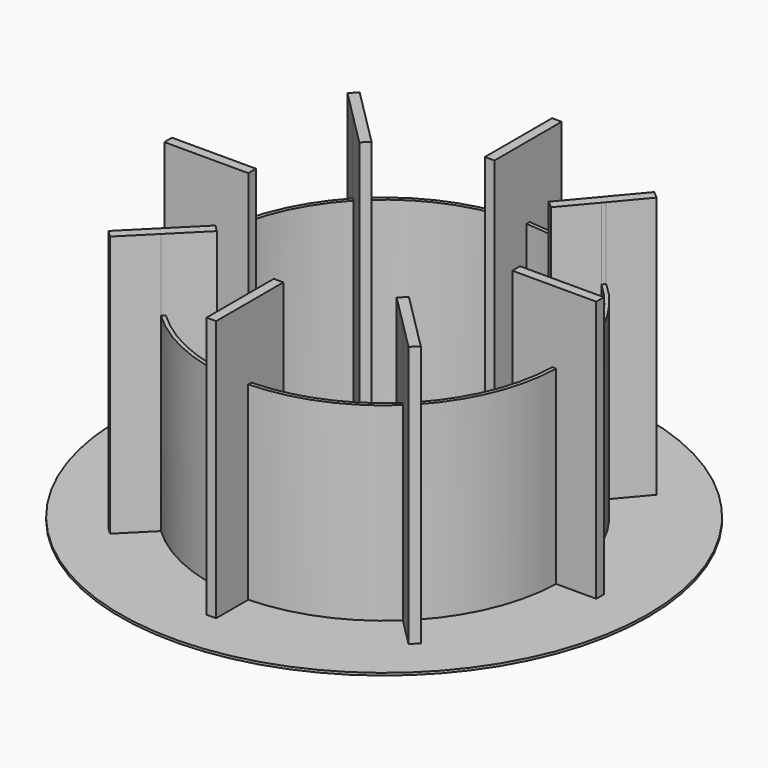
from build123d import *

# Parameters (mm, degrees)
F0_R     = 110
F1_DEPTH = 1
F0_R_2   = 7.5
F2_DEPTH = 110
F3_DEPTH = 80


with BuildPart() as f1:
    # F0 (on Top) → F1 (new body)
    with BuildSketch(Plane.XY):
        Circle(F0_R)
        with BuildLine():
            Line((-90, 2), (-73.2727097902, 2))
            ThreePointArc((-73.2727097902, 2), (-67.7203697331, 28.0506955924), (-53.2258435309, 50.3974164062))
            Line((-53.2258435309, 50.3974164062), (-65.0538238692, 62.2253967444))
            Line((-65.0538238692, 62.2253967444), (-62.2253967444, 65.0538238692))
            Line((-62.2253967444, 65.0538238692), (-50.3974164062, 53.2258435309))
            ThreePointArc((-50.3974164062, 53.2258435309), (-28.0506955924, 67.7203697331), (-2, 73.2727097902))
            Line((-2, 73.2727097902), (-2, 90))
            Line((-2, 90), (2, 90))
            Line((2, 90), (2, 73.2727097902))
            ThreePointArc((2, 73.2727097902), (25.1459027822, 68.8518233111), (45.6930285955, 57.3152435027))
            Line((45.6930285955, 57.3152435027), (56.4733154171, 70.105382431))
            Line((56.4733154171, 70.105382431), (59.5318237034, 67.5274904506))
            Line((59.5318237034, 67.5274904506), (48.7515368817, 54.7373515223))
            ThreePointArc((48.7515368817, 54.7373515223), (66.4664295367, 30.904752784), (73.2727097902, 2))
            Line((73.2727097902, 2), (90, 2))
            Line((90, 2), (90, -2))
            Line((90, -2), (73.2727097902, -2))
            ThreePointArc((73.2727097902, -2), (67.7203697331, -28.0506955924), (53.2258435309, -50.3974164062))
            Line((53.2258435309, -50.3974164062), (65.0538238692, -62.2253967444))
            Line((65.0538238692, -62.2253967444), (62.2253967444, -65.0538238692))
            Line((62.2253967444, -65.0538238692), (50.3974164062, -53.2258435309))
            ThreePointArc((50.3974164062, -53.2258435309), (28.0506955924, -67.7203697331), (2, -73.2727097902))
            Line((2, -73.2727097902), (2, -90))
            Line((2, -90), (-2, -90))
            Line((-2, -90), (-2, -73.2727097902))
            ThreePointArc((-2, -73.2727097902), (-28.0506955924, -67.7203697331), (-50.3974164062, -53.2258435309))
            Line((-50.3974164062, -53.2258435309), (-62.2253967444, -65.0538238692))
            Line((-62.2253967444, -65.0538238692), (-65.0538238692, -62.2253967444))
            Line((-65.0538238692, -62.2253967444), (-53.2258435309, -50.3974164062))
            ThreePointArc((-53.2258435309, -50.3974164062), (-67.7203697331, -28.0506955924), (-73.2727097902, -2))
            Line((-73.2727097902, -2), (-90, -2))
            Line((-90, -2), (-90, 2))
        make_face(mode=Mode.SUBTRACT)
    extrude(amount=F1_DEPTH)



with BuildPart() as f1b:
    # F0 (on Top) → F1, piece 2 (new body)
    with BuildSketch(Plane.XY):
        with BuildLine():
            Line((-71.6721005692, 2), (-55, 2))
            Line((-55, 2), (-55, -2))
            Line((-55, -2), (-71.6721005692, -2))
            ThreePointArc((-71.6721005692, -2), (-66.2421624811, -27.4384021006), (-52.0940418967, -49.265614772))
            Line((-52.0940418967, -49.265614772), (-40.3050865276, -37.4766594029))
            Line((-40.3050865276, -37.4766594029), (-37.4766594029, -40.3050865276))
            Line((-37.4766594029, -40.3050865276), (-49.265614772, -52.0940418967))
            ThreePointArc((-49.265614772, -52.0940418967), (-27.4384021006, -66.2421624811), (-2, -71.6721005692))
            Line((-2, -71.6721005692), (-2, -55))
            Line((-2, -55), (2, -55))
            Line((2, -55), (2, -71.6721005692))
            ThreePointArc((2, -71.6721005692), (27.4384021006, -66.2421624811), (49.265614772, -52.0940418967))
            Line((49.265614772, -52.0940418967), (37.4766594029, -40.3050865276))
            Line((37.4766594029, -40.3050865276), (40.3050865276, -37.4766594029))
            Line((40.3050865276, -37.4766594029), (52.0940418967, -49.265614772))
            ThreePointArc((52.0940418967, -49.265614772), (66.2421624811, -27.4384021006), (71.6721005692, -2))
            Line((71.6721005692, -2), (55, -2))
            Line((55, -2), (55, 2))
            Line((55, 2), (71.6721005692, 2))
            ThreePointArc((71.6721005692, 2), (65.0155934213, 30.2301606359), (47.719987463, 53.5134823809))
            Line((47.719987463, 53.5134823809), (36.9752688744, 40.7655429458))
            Line((36.9752688744, 40.7655429458), (33.9167605881, 43.3434349263))
            Line((33.9167605881, 43.3434349263), (44.6614791768, 56.0913743613))
            ThreePointArc((44.6614791768, 56.0913743613), (24.597015409, 67.3489185731), (2, 71.6721005692))
            Line((2, 71.6721005692), (2, 55))
            Line((2, 55), (-2, 55))
            Line((-2, 55), (-2, 71.6721005692))
            ThreePointArc((-2, 71.6721005692), (-27.4384021006, 66.2421624811), (-49.265614772, 52.0940418967))
            Line((-49.265614772, 52.0940418967), (-37.4766594029, 40.3050865276))
            Line((-37.4766594029, 40.3050865276), (-40.3050865276, 37.4766594029))
            Line((-40.3050865276, 37.4766594029), (-52.0940418967, 49.265614772))
            ThreePointArc((-52.0940418967, 49.265614772), (-66.2421624811, 27.4384021006), (-71.6721005692, 2))
        make_face()
        Circle(F0_R_2, mode=Mode.SUBTRACT)
    extrude(amount=F1_DEPTH)


with BuildPart() as f1_1:
    add(f1.part)

    add(f1b.part)  # F2 merges F1b
    # F0 (on Top) → F2 (join)
    with BuildSketch(Plane.XY):
        with BuildLine():
            Line((-55, -2), (-55, 2))
            Line((-55, 2), (-71.6721005692, 2))
            ThreePointArc((-71.6721005692, 2), (-71.7, 0), (-71.6721005692, -2))
            Line((-71.6721005692, -2), (-55, -2))
        make_face()
        with BuildLine():
            ThreePointArc((-71.6721005692, -2), (-71.7, 0), (-71.6721005692, 2))
            Line((-71.6721005692, 2), (-73.2727097902, 2))
            ThreePointArc((-73.2727097902, 2), (-73.3, 0), (-73.2727097902, -2))
            Line((-73.2727097902, -2), (-71.6721005692, -2))
        make_face()
        with BuildLine():
            ThreePointArc((-73.2727097902, -2), (-73.3, 0), (-73.2727097902, 2))
            Line((-73.2727097902, 2), (-90, 2))
            Line((-90, 2), (-90, -2))
            Line((-90, -2), (-73.2727097902, -2))
        make_face()
        with BuildLine():
            ThreePointArc((-49.265614772, 52.0940418967), (-50.6995562111, 50.6995562111), (-52.0940418967, 49.265614772))
            Line((-52.0940418967, 49.265614772), (-40.3050865276, 37.4766594029))
            Line((-40.3050865276, 37.4766594029), (-37.4766594029, 40.3050865276))
            Line((-37.4766594029, 40.3050865276), (-49.265614772, 52.0940418967))
        make_face()
        with BuildLine():
            Line((-53.2258435309, 50.3974164062), (-52.0940418967, 49.265614772))
            ThreePointArc((-52.0940418967, 49.265614772), (-50.6995562111, 50.6995562111), (-49.265614772, 52.0940418967))
            Line((-49.265614772, 52.0940418967), (-50.3974164062, 53.2258435309))
            ThreePointArc((-50.3974164062, 53.2258435309), (-51.830927061, 51.830927061), (-53.2258435309, 50.3974164062))
        make_face()
        with BuildLine():
            Line((-65.0538238692, 62.2253967444), (-53.2258435309, 50.3974164062))
            ThreePointArc((-53.2258435309, 50.3974164062), (-51.830927061, 51.830927061), (-50.3974164062, 53.2258435309))
            Line((-50.3974164062, 53.2258435309), (-62.2253967444, 65.0538238692))
            Line((-62.2253967444, 65.0538238692), (-65.0538238692, 62.2253967444))
        make_face()
        with BuildLine():
            ThreePointArc((2, 71.6721005692), (0, 71.7), (-2, 71.6721005692))
            Line((-2, 71.6721005692), (-2, 55))
            Line((-2, 55), (2, 55))
            Line((2, 55), (2, 71.6721005692))
        make_face()
        with BuildLine():
            Line((-2, 73.2727097902), (-2, 71.6721005692))
            ThreePointArc((-2, 71.6721005692), (0, 71.7), (2, 71.6721005692))
            Line((2, 71.6721005692), (2, 73.2727097902))
            ThreePointArc((2, 73.2727097902), (0, 73.3), (-2, 73.2727097902))
        make_face()
        with BuildLine():
            Line((-2, 90), (-2, 73.2727097902))
            ThreePointArc((-2, 73.2727097902), (0, 73.3), (2, 73.2727097902))
            Line((2, 73.2727097902), (2, 90))
            Line((2, 90), (-2, 90))
        make_face()
        with BuildLine():
            ThreePointArc((47.719987463, 53.5134823809), (46.2087137496, 54.8237610312), (44.6614791768, 56.0913743613))
            Line((44.6614791768, 56.0913743613), (33.9167605881, 43.3434349263))
            Line((33.9167605881, 43.3434349263), (36.9752688744, 40.7655429458))
            Line((36.9752688744, 40.7655429458), (47.719987463, 53.5134823809))
        make_face()
        with BuildLine():
            Line((45.6930285955, 57.3152435027), (44.6614791768, 56.0913743613))
            ThreePointArc((44.6614791768, 56.0913743613), (46.2087137496, 54.8237610312), (47.719987463, 53.5134823809))
            Line((47.719987463, 53.5134823809), (48.7515368817, 54.7373515223))
            ThreePointArc((48.7515368817, 54.7373515223), (47.2398705418, 56.0471643457), (45.6930285955, 57.3152435027))
        make_face()
        with BuildLine():
            Line((56.4733154171, 70.105382431), (45.6930285955, 57.3152435027))
            ThreePointArc((45.6930285955, 57.3152435027), (47.2398705418, 56.0471643457), (48.7515368817, 54.7373515223))
            Line((48.7515368817, 54.7373515223), (59.5318237034, 67.5274904506))
            Line((59.5318237034, 67.5274904506), (56.4733154171, 70.105382431))
        make_face()
        with BuildLine():
            ThreePointArc((71.7, 0), (71.693024803, 1.0000972925), (71.6721005692, 2))
            Line((71.6721005692, 2), (55, 2))
            Line((55, 2), (55, -2))
            Line((55, -2), (71.6721005692, -2))
            ThreePointArc((71.6721005692, -2), (71.693024803, -1.0000972925), (71.7, 0))
        make_face()
        with BuildLine():
            Line((73.2727097902, 2), (71.6721005692, 2))
            ThreePointArc((71.6721005692, 2), (71.693024803, 1.0000972925), (71.7, 0))
            ThreePointArc((71.7, 0), (71.693024803, -1.0000972925), (71.6721005692, -2))
            Line((71.6721005692, -2), (73.2727097902, -2))
            ThreePointArc((73.2727097902, -2), (73.29317713, -1.0000930901), (73.3, 0))
            ThreePointArc((73.3, 0), (73.29317713, 1.0000930901), (73.2727097902, 2))
        make_face()
        with BuildLine():
            Line((90, 2), (73.2727097902, 2))
            ThreePointArc((73.2727097902, 2), (73.29317713, 1.0000930901), (73.3, 0))
            ThreePointArc((73.3, 0), (73.29317713, -1.0000930901), (73.2727097902, -2))
            Line((73.2727097902, -2), (90, -2))
            Line((90, -2), (90, 2))
        make_face()
        with BuildLine():
            Line((37.4766594029, -40.3050865276), (49.265614772, -52.0940418967))
            ThreePointArc((49.265614772, -52.0940418967), (50.6995562111, -50.6995562111), (52.0940418967, -49.265614772))
            Line((52.0940418967, -49.265614772), (40.3050865276, -37.4766594029))
            Line((40.3050865276, -37.4766594029), (37.4766594029, -40.3050865276))
        make_face()
        with BuildLine():
            ThreePointArc((52.0940418967, -49.265614772), (50.6995562111, -50.6995562111), (49.265614772, -52.0940418967))
            Line((49.265614772, -52.0940418967), (50.3974164062, -53.2258435309))
            ThreePointArc((50.3974164062, -53.2258435309), (51.830927061, -51.830927061), (53.2258435309, -50.3974164062))
            Line((53.2258435309, -50.3974164062), (52.0940418967, -49.265614772))
        make_face()
        with BuildLine():
            ThreePointArc((53.2258435309, -50.3974164062), (51.830927061, -51.830927061), (50.3974164062, -53.2258435309))
            Line((50.3974164062, -53.2258435309), (62.2253967444, -65.0538238692))
            Line((62.2253967444, -65.0538238692), (65.0538238692, -62.2253967444))
            Line((65.0538238692, -62.2253967444), (53.2258435309, -50.3974164062))
        make_face()
        with BuildLine():
            Line((-2, -55), (-2, -71.6721005692))
            ThreePointArc((-2, -71.6721005692), (0, -71.7), (2, -71.6721005692))
            Line((2, -71.6721005692), (2, -55))
            Line((2, -55), (-2, -55))
        make_face()
        with BuildLine():
            ThreePointArc((2, -71.6721005692), (0, -71.7), (-2, -71.6721005692))
            Line((-2, -71.6721005692), (-2, -73.2727097902))
            ThreePointArc((-2, -73.2727097902), (0, -73.3), (2, -73.2727097902))
            Line((2, -73.2727097902), (2, -71.6721005692))
        make_face()
        with BuildLine():
            ThreePointArc((2, -73.2727097902), (0, -73.3), (-2, -73.2727097902))
            Line((-2, -73.2727097902), (-2, -90))
            Line((-2, -90), (2, -90))
            Line((2, -90), (2, -73.2727097902))
        make_face()
        with BuildLine():
            Line((-40.3050865276, -37.4766594029), (-52.0940418967, -49.265614772))
            ThreePointArc((-52.0940418967, -49.265614772), (-50.6995562111, -50.6995562111), (-49.265614772, -52.0940418967))
            Line((-49.265614772, -52.0940418967), (-37.4766594029, -40.3050865276))
            Line((-37.4766594029, -40.3050865276), (-40.3050865276, -37.4766594029))
        make_face()
        with BuildLine():
            ThreePointArc((-49.265614772, -52.0940418967), (-50.6995562111, -50.6995562111), (-52.0940418967, -49.265614772))
            Line((-52.0940418967, -49.265614772), (-53.2258435309, -50.3974164062))
            ThreePointArc((-53.2258435309, -50.3974164062), (-51.830927061, -51.830927061), (-50.3974164062, -53.2258435309))
            Line((-50.3974164062, -53.2258435309), (-49.265614772, -52.0940418967))
        make_face()
        with BuildLine():
            ThreePointArc((-50.3974164062, -53.2258435309), (-51.830927061, -51.830927061), (-53.2258435309, -50.3974164062))
            Line((-53.2258435309, -50.3974164062), (-65.0538238692, -62.2253967444))
            Line((-65.0538238692, -62.2253967444), (-62.2253967444, -65.0538238692))
            Line((-62.2253967444, -65.0538238692), (-50.3974164062, -53.2258435309))
        make_face()
    extrude(amount=F2_DEPTH)

    # F0 (on Top) → F3 (join)
    with BuildSketch(Plane.XY):
        with BuildLine():
            Line((-73.2727097902, 2), (-71.6721005692, 2))
            ThreePointArc((-71.6721005692, 2), (-66.2421624811, 27.4384021006), (-52.0940418967, 49.265614772))
            Line((-52.0940418967, 49.265614772), (-53.2258435309, 50.3974164062))
            ThreePointArc((-53.2258435309, 50.3974164062), (-67.7203697331, 28.0506955924), (-73.2727097902, 2))
        make_face()
        with BuildLine():
            Line((-50.3974164062, 53.2258435309), (-49.265614772, 52.0940418967))
            ThreePointArc((-49.265614772, 52.0940418967), (-27.4384021006, 66.2421624811), (-2, 71.6721005692))
            Line((-2, 71.6721005692), (-2, 73.2727097902))
            ThreePointArc((-2, 73.2727097902), (-28.0506955924, 67.7203697331), (-50.3974164062, 53.2258435309))
        make_face()
        with BuildLine():
            Line((2, 73.2727097902), (2, 71.6721005692))
            ThreePointArc((2, 71.6721005692), (24.597015409, 67.3489185731), (44.6614791768, 56.0913743613))
            Line((44.6614791768, 56.0913743613), (45.6930285955, 57.3152435027))
            ThreePointArc((45.6930285955, 57.3152435027), (25.1459027822, 68.8518233111), (2, 73.2727097902))
        make_face()
        with BuildLine():
            Line((48.7515368817, 54.7373515223), (47.719987463, 53.5134823809))
            ThreePointArc((47.719987463, 53.5134823809), (65.0155934213, 30.2301606359), (71.6721005692, 2))
            Line((71.6721005692, 2), (73.2727097902, 2))
            ThreePointArc((73.2727097902, 2), (66.4664295367, 30.904752784), (48.7515368817, 54.7373515223))
        make_face()
        with BuildLine():
            ThreePointArc((71.6721005692, -2), (66.2421624811, -27.4384021006), (52.0940418967, -49.265614772))
            Line((52.0940418967, -49.265614772), (53.2258435309, -50.3974164062))
            ThreePointArc((53.2258435309, -50.3974164062), (67.7203697331, -28.0506955924), (73.2727097902, -2))
            Line((73.2727097902, -2), (71.6721005692, -2))
        make_face()
        with BuildLine():
            ThreePointArc((49.265614772, -52.0940418967), (27.4384021006, -66.2421624811), (2, -71.6721005692))
            Line((2, -71.6721005692), (2, -73.2727097902))
            ThreePointArc((2, -73.2727097902), (28.0506955924, -67.7203697331), (50.3974164062, -53.2258435309))
            Line((50.3974164062, -53.2258435309), (49.265614772, -52.0940418967))
        make_face()
        with BuildLine():
            ThreePointArc((-2, -71.6721005692), (-27.4384021006, -66.2421624811), (-49.265614772, -52.0940418967))
            Line((-49.265614772, -52.0940418967), (-50.3974164062, -53.2258435309))
            ThreePointArc((-50.3974164062, -53.2258435309), (-28.0506955924, -67.7203697331), (-2, -73.2727097902))
            Line((-2, -73.2727097902), (-2, -71.6721005692))
        make_face()
        with BuildLine():
            ThreePointArc((-52.0940418967, -49.265614772), (-66.2421624811, -27.4384021006), (-71.6721005692, -2))
            Line((-71.6721005692, -2), (-73.2727097902, -2))
            ThreePointArc((-73.2727097902, -2), (-67.7203697331, -28.0506955924), (-53.2258435309, -50.3974164062))
            Line((-53.2258435309, -50.3974164062), (-52.0940418967, -49.265614772))
        make_face()
    extrude(amount=F3_DEPTH)


solid = f1_1.part
